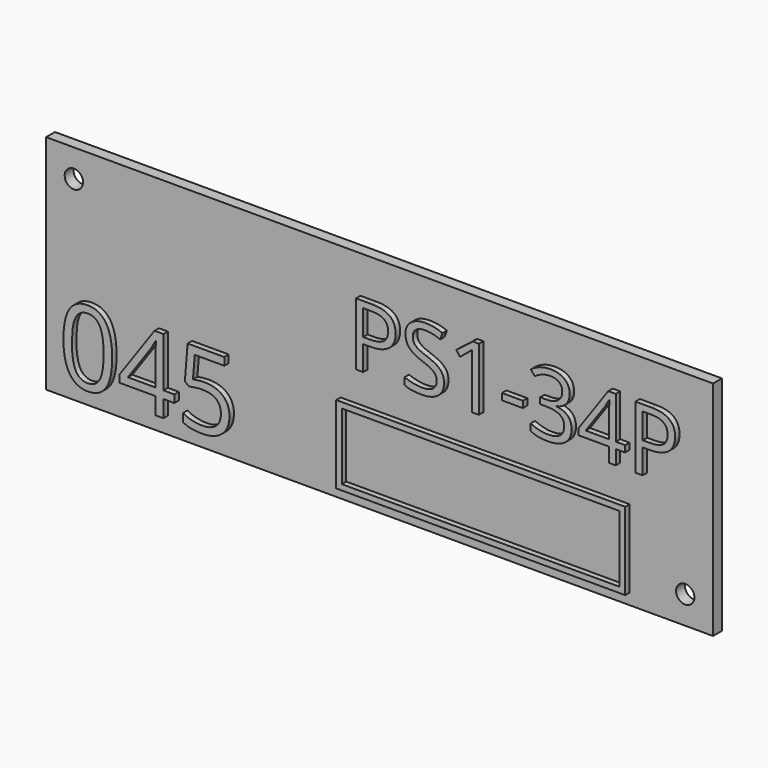
from build123d import *

# Parameters (mm, degrees)
F0_W         = 120
F0_H         = 40
F1_DEPTH     = 2
F3_D         = 3.3
F4_TEXT_SIZE = 15.7752033522
F5_DEPTH     = 1
F6_TEXT_SIZE = 18.5776487663
F7_DEPTH     = 1
F8_W         = 52
F8_H         = 14
F8_W_2       = 49.99999962
F8_H_2       = 11.99999962
F9_DEPTH     = 1


# Not quite as in the source:
# - Text() gives the source's letters only with a copy of the font that has no kerning and outlines rounded to 1/6400 em; it was checked with that copy


with BuildPart() as f1:
    # F0 (on Front) → F1 (new body)
    with BuildSketch(Plane.XZ):
        Rectangle(F0_W, F0_H)
    extrude(amount=F1_DEPTH)

    # F3 (through all)
    with Locations(Plane.XZ.offset(2)):
        with Locations((-55, 15), (55, -15)):
            Hole(F3_D / 2)

    # F4 (on face) → F5 (join)
    with BuildSketch(Plane.XZ.offset(2)):
        with Locations((-5, 2)):
            Text('PS1-34P', F4_TEXT_SIZE, font='Open Sans', text_align=(TextAlign.LEFT, TextAlign.BOTTOM))
    extrude(amount=F5_DEPTH)

    # F6 (on face) → F7 (join)
    with BuildSketch(Plane.XZ.offset(2)):
        with Locations((-57, -17)):
            Text('045', F6_TEXT_SIZE, font='Open Sans', text_align=(TextAlign.LEFT, TextAlign.BOTTOM))
    extrude(amount=F7_DEPTH)

    # F8 (on face) → F9 (join)
    with BuildSketch(Plane.XZ.offset(2)):
        with Locations((19, -11)):
            Rectangle(F8_W, F8_H)
        with Locations((19, -11)):
            Rectangle(F8_W_2, F8_H_2, mode=Mode.SUBTRACT)
    extrude(amount=F9_DEPTH)


solid = f1.part
